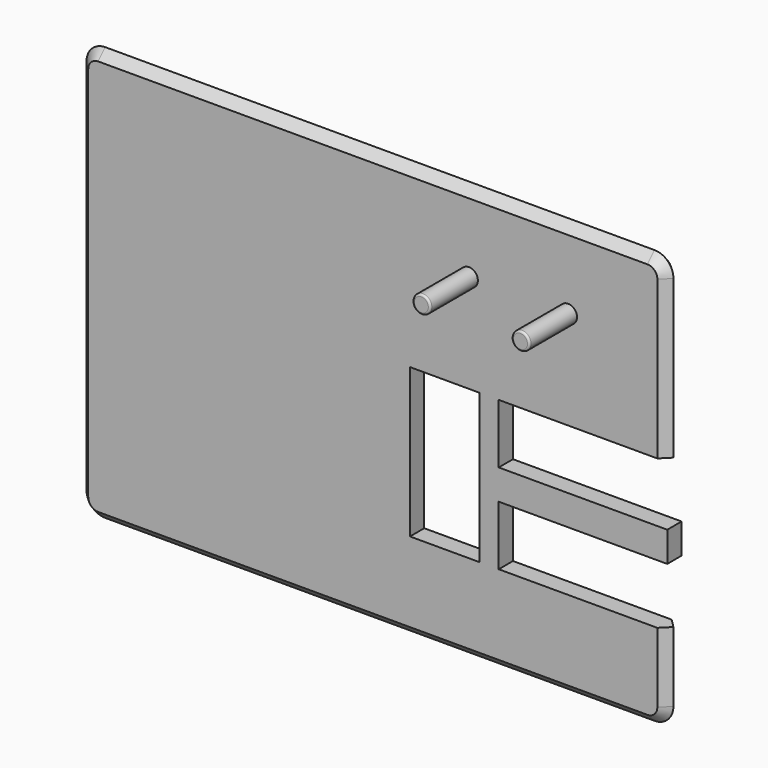
from build123d import *

# Parameters (mm, degrees)
F1_DEPTH      = 9
F2_R          = 4.5
F3_DEPTH      = 30
F4_W          = 85
F4_H          = 30
F5_DEPTH      = 25
F6_W          = 85
F6_H          = 30
F7_DEPTH      = 25
F9_R          = 1
F10_T1_DEPTH  = 277
F10_T3_DEPTH  = 190
F10_T5_DEPTH  = 48.1001500805
F10_T7_DEPTH  = 92.4223044172
F10_T10_ANGLE = 90
F10_T12_ANGLE = 90
F10_T14_ANGLE = 90
F10_T16_ANGLE = 90
F10_T18_ANGLE = 90
F10_T20_ANGLE = 90
F10_T22_ANGLE = 90
F10_T24_ANGLE = 90
F8_W          = 35
F8_H          = 75.194375382
F11_DEPTH     = 25


# Not quite as in the source:
# - a fillet or chamfer that OpenCascade refuses, or shapes differently, is made with other operations: its cross-section is extruded or revolved along the edge and cut away or added


with BuildPart() as f1:
    # F0 (on Front) → F1 (new body)
    with BuildSketch(Plane.XZ):
        with BuildLine():
            Line((131.9335396439, -4.1335214776), (-145.0664603561, -4.1335214776))
            ThreePointArc((-145.0664603561, -4.1335214776), (-152.137528168, -7.0624536657), (-155.0664603561, -14.1335214776))
            Line((-155.0664603561, -14.1335214776), (-155.0664603561, -204.1335214776))
            ThreePointArc((-155.0664603561, -204.1335214776), (-152.137528168, -211.2045892894), (-145.0664603561, -214.1335214776))
            Line((-145.0664603561, -214.1335214776), (131.9335396439, -214.1335214776))
            ThreePointArc((131.9335396439, -214.1335214776), (139.0046074557, -211.2045892894), (141.9335396439, -204.1335214776))
            Line((141.9335396439, -204.1335214776), (141.9335396439, -14.1335214776))
            ThreePointArc((141.9335396439, -14.1335214776), (139.0046074557, -7.0624536657), (131.9335396439, -4.1335214776))
        make_face()
    extrude(amount=F1_DEPTH)

    # F2 (on face) → F3 (join)
    with BuildSketch(Plane.XZ.offset(9)):
        with Locations((41.9335396439, -44.1335214776)):
            Circle(F2_R)
        with Locations((91.9335396439, -44.1335214776)):
            Circle(F2_R)
    extrude(amount=F3_DEPTH)

    # F4 (on face) → F5 (cut)
    with BuildSketch(Plane.XZ.offset(9)):
        with Locations((99.4335396439, -108.6974109549)):
            Rectangle(F4_W, F4_H)
    extrude(amount=-F5_DEPTH, mode=Mode.SUBTRACT)

    # F6 (on face) → F7 (cut)
    with BuildSketch(Plane.XZ.offset(9)):
        with Locations((99.4335396439, -153.8917863369)):
            Rectangle(F6_W, F6_H)
    extrude(amount=-F7_DEPTH, mode=Mode.SUBTRACT)

    # F9
    f9_edges = [f1.edges().sort_by_distance(p)[0] for p in [
        (37.43354, -39, -44.133521),
        (87.43354, -39, -44.133521),
    ]]
    fillet(f9_edges, radius=F9_R)

    # F10: chamfer of 5 on 2 edges, made by hand

    # F10_s2 → F10_t1 (cut)
    with BuildSketch(Plane.YZ.offset(-145.0664603561)):
        Polygon((-9, -9.1335214776), (-4, -4.1335214776), (-9, -4.1335214776), align=None)
        Polygon((-5, -4.1335214776), (0, -9.1335214776), (0, -4.1335214776), align=None)
        Polygon((-5, -214.1335214776), (0, -209.1335214776), (0, -214.1335214776), align=None)
        Polygon((-9, -209.1335214776), (-4, -214.1335214776), (-9, -214.1335214776), align=None)
    extrude(amount=F10_T1_DEPTH, mode=Mode.SUBTRACT)

    # F10_s4 → F10_t3 (cut)
    with BuildSketch(Plane.XY.offset(-204.1335214776)):
        Polygon((-155.0664603561, -5), (-150.0664603561, 0), (-155.0664603561, 0), align=None)
        Polygon((-150.0664603561, -9), (-155.0664603561, -4), (-155.0664603561, -9), align=None)
    extrude(amount=F10_T3_DEPTH, mode=Mode.SUBTRACT)

    # F10_s6 → F10_t5 (cut)
    with BuildSketch(Plane.XY.offset(-204.1335214776)):
        Polygon((141.9335396439, -5), (136.9335396439, 0), (141.9335396439, 0), align=None)
        Polygon((136.9335396439, -9), (141.9335396439, -4), (141.9335396439, -9), align=None)
    extrude(amount=F10_T5_DEPTH, mode=Mode.SUBTRACT)

    # F10_s8 → F10_t7 (cut)
    with BuildSketch(Plane.XY.offset(-106.5558258947)):
        Polygon((141.9335396439, -5), (136.9335396439, 0), (141.9335396439, 0), align=None)
        Polygon((136.9335396439, -9), (141.9335396439, -4), (141.9335396439, -9), align=None)
    extrude(amount=F10_T7_DEPTH, mode=Mode.SUBTRACT)

    # F10_s9 → F10_t10 (revolve, cut)
    with BuildSketch(Plane.XY.offset(-14.1335214776)):
        Polygon((141.9335396439, -5), (136.9335396439, 0), (141.9335396439, 0), align=None)
    revolve(axis=Axis((131.9335396439, 0, -14.1335214776), (0, -1, 0)), revolution_arc=F10_T10_ANGLE, mode=Mode.SUBTRACT)

    # F10_s11 → F10_t12 (revolve, cut)
    with BuildSketch(Plane.YZ.offset(-145.0664603561)):
        Polygon((-5, -4.1335214776), (0, -9.1335214776), (0, -4.1335214776), align=None)
    revolve(axis=Axis((-145.0664603561, 0, -14.1335214776), (0, -1, 0)), revolution_arc=F10_T12_ANGLE, mode=Mode.SUBTRACT)

    # F10_s13 → F10_t14 (revolve, cut)
    with BuildSketch(Plane.XY.offset(-204.1335214776)):
        Polygon((-155.0664603561, -5), (-150.0664603561, 0), (-155.0664603561, 0), align=None)
    revolve(axis=Axis((-145.0664603561, 0, -204.1335214776), (0, -1, 0)), revolution_arc=F10_T14_ANGLE, mode=Mode.SUBTRACT)

    # F10_s15 → F10_t16 (revolve, cut)
    with BuildSketch(Plane.YZ.offset(131.9335396439)):
        Polygon((-5, -214.1335214776), (0, -209.1335214776), (0, -214.1335214776), align=None)
    revolve(axis=Axis((131.9335396439, 0, -204.1335214776), (0, -1, 0)), revolution_arc=F10_T16_ANGLE, mode=Mode.SUBTRACT)

    # F10_s17 → F10_t18 (revolve, cut)
    with BuildSketch(Plane.XY.offset(-14.1335214776)):
        Polygon((136.9335396439, -9), (141.9335396439, -4), (141.9335396439, -9), align=None)
    revolve(axis=Axis((131.9335396439, -9, -14.1335214776), (0, -1, 0)), revolution_arc=F10_T18_ANGLE, mode=Mode.SUBTRACT)

    # F10_s19 → F10_t20 (revolve, cut)
    with BuildSketch(Plane.YZ.offset(-145.0664603561)):
        Polygon((-9, -9.1335214776), (-4, -4.1335214776), (-9, -4.1335214776), align=None)
    revolve(axis=Axis((-145.0664603561, -9, -14.1335214776), (0, -1, 0)), revolution_arc=F10_T20_ANGLE, mode=Mode.SUBTRACT)

    # F10_s21 → F10_t22 (revolve, cut)
    with BuildSketch(Plane.XY.offset(-204.1335214776)):
        Polygon((-150.0664603561, -9), (-155.0664603561, -4), (-155.0664603561, -9), align=None)
    revolve(axis=Axis((-145.0664603561, -9, -204.1335214776), (0, -1, 0)), revolution_arc=F10_T22_ANGLE, mode=Mode.SUBTRACT)

    # F10_s23 → F10_t24 (revolve, cut)
    with BuildSketch(Plane.YZ.offset(131.9335396439)):
        Polygon((-9, -209.1335214776), (-4, -214.1335214776), (-9, -214.1335214776), align=None)
    revolve(axis=Axis((131.9335396439, -9, -204.1335214776), (0, -1, 0)), revolution_arc=F10_T24_ANGLE, mode=Mode.SUBTRACT)

    # F8 (on face) → F11 (cut)
    with BuildSketch(Plane.XZ.offset(9)):
        with Locations((29.6793225408, -131.2945986459)):
            Rectangle(F8_W, F8_H)
    extrude(amount=-F11_DEPTH, mode=Mode.SUBTRACT)


solid = f1.part
